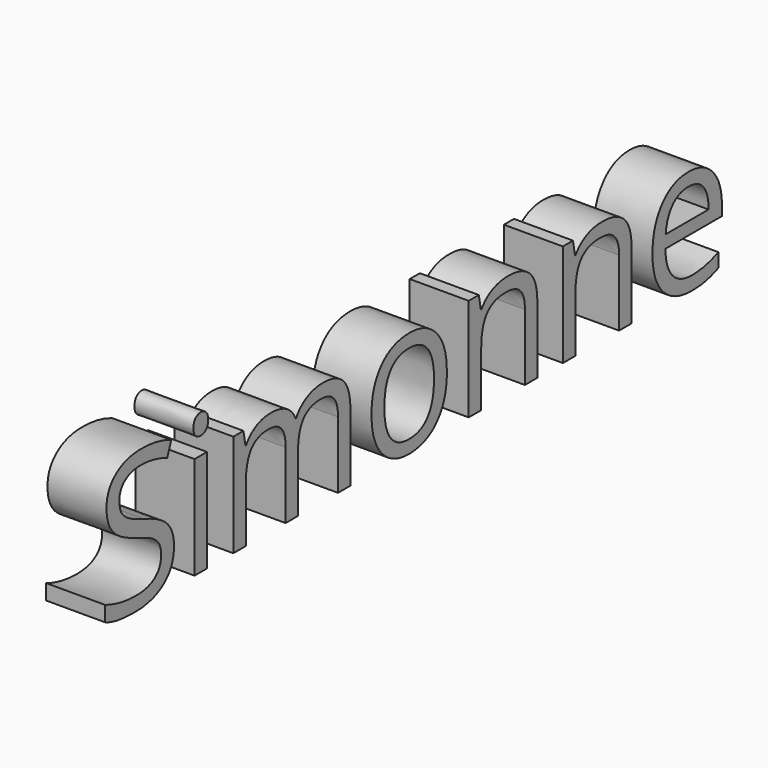
from build123d import *

# Parameters (mm, degrees)
F0_TEXT_SIZE = 82.5870083645
F1_DEPTH     = 25.4


# Not quite as in the source:
# - Text() gives the source's letters only with a copy of the font that has no kerning and outlines rounded to 1/6400 em; it was checked with that copy


with BuildPart() as f1:
    # F0 (on Right) → F1 (new body)
    with BuildSketch(Plane.YZ):
        with Locations((-153.6733312532, -32.0734791458)):
            Text('Simonne', F0_TEXT_SIZE, font='Open Sans', text_align=(TextAlign.LEFT, TextAlign.BOTTOM))
    extrude(amount=F1_DEPTH)


solid = f1.part
